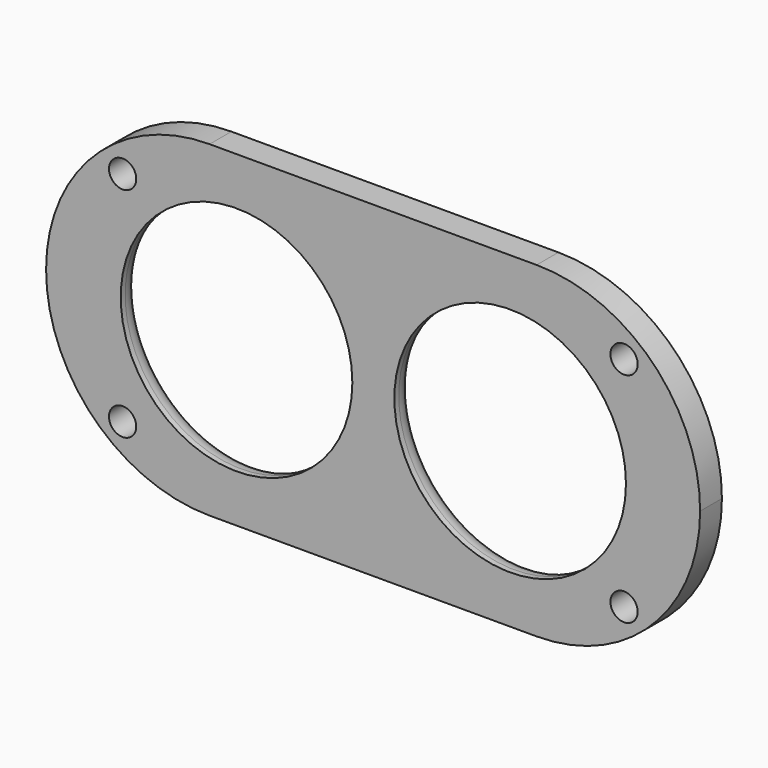
from build123d import *

# Parameters (mm, degrees)
F0_R     = 3.175
F1_DEPTH = 6.35
F2_DEPTH = 6.35
F4_R     = 26.9875
F5_DEPTH = 25.4


# Not quite as in the source:
# - a fillet or chamfer that OpenCascade refuses, or shapes differently, is made with other operations: its cross-section is extruded or revolved along the edge and cut away or added


with BuildPart() as f1:
    # F0 (on Front) → F1 (new body)
    with BuildSketch(Plane.XZ):
        with BuildLine():
            ThreePointArc((-76.2542010712, 0), (-65.0949694344, -26.9407683632), (-38.1542010712, -38.1))
            Line((-38.1542010712, -38.1), (38.0457989288, -38.1))
            ThreePointArc((38.0457989288, -38.1), (64.986567292, -26.9407683632), (76.1457989288, 0))
            ThreePointArc((76.1457989288, 0), (64.986567292, 26.9407683632), (38.0457989288, 38.1))
            Line((38.0457989288, 38.1), (-38.1542010712, 38.1))
            ThreePointArc((-38.1542010712, 38.1), (-65.0949694344, 26.9407683632), (-76.2542010712, 0))
        make_face()
        with Locations((-58.42, -25.4)):
            Circle(F0_R, mode=Mode.SUBTRACT)
        with Locations((58.42, -25.4)):
            Circle(F0_R, mode=Mode.SUBTRACT)
        with Locations((-58.42, 25.4)):
            Circle(F0_R, mode=Mode.SUBTRACT)
        with BuildLine():
            ThreePointArc((-31.75, -31.75), (-63.5, 0), (-31.75, 31.75))
            Line((-31.75, 31.75), (31.75, 31.75))
            ThreePointArc((31.75, 31.75), (63.5, 0), (31.75, -31.75))
            Line((31.75, -31.75), (-31.75, -31.75))
        make_face(mode=Mode.SUBTRACT)
        with Locations((58.42, 25.4)):
            Circle(F0_R, mode=Mode.SUBTRACT)
    extrude(amount=F1_DEPTH)

    # F0 (on Front) → F2 (join)
    with BuildSketch(Plane.XZ):
        with BuildLine():
            Line((31.75, 31.75), (-31.75, 31.75))
            ThreePointArc((-31.75, 31.75), (-63.5, 0), (-31.75, -31.75))
            Line((-31.75, -31.75), (31.75, -31.75))
            ThreePointArc((31.75, -31.75), (63.5, 0), (31.75, 31.75))
        make_face()
    extrude(amount=F2_DEPTH)

    # F4 (on face) → F5 (cut)
    with BuildSketch(Plane.XZ.offset(6.35)):
        with Locations((-31.877, 0)):
            Circle(F4_R)
        with Locations((31.877, 0)):
            Circle(F4_R)
    extrude(amount=-F5_DEPTH, mode=Mode.SUBTRACT)

    # F6: fillet of radius 5.08 on 2 edges, made by hand

    # F6_s1 → F6_t2 (revolve, cut)
    with BuildSketch(Plane.XY):
        with BuildLine():
            ThreePointArc((63.9445, 0), (60.3523975516, -1.4878975516), (58.8645, -5.08))
            Line((58.8645, -5.08), (58.8645, 0))
            Line((58.8645, 0), (63.9445, 0))
        make_face()
    revolve(axis=Axis((31.877, 0, 0), (0, -1, 0)), mode=Mode.SUBTRACT)

    # F6_s3 → F6_t4 (revolve, cut)
    with BuildSketch(Plane.XY):
        with BuildLine():
            ThreePointArc((0.1905, 0), (-3.4016024484, -1.4878975516), (-4.8895, -5.08))
            Line((-4.8895, -5.08), (-4.8895, 0))
            Line((-4.8895, 0), (0.1905, 0))
        make_face()
    revolve(axis=Axis((-31.877, 0, 0), (0, -1, 0)), mode=Mode.SUBTRACT)


solid = f1.part
